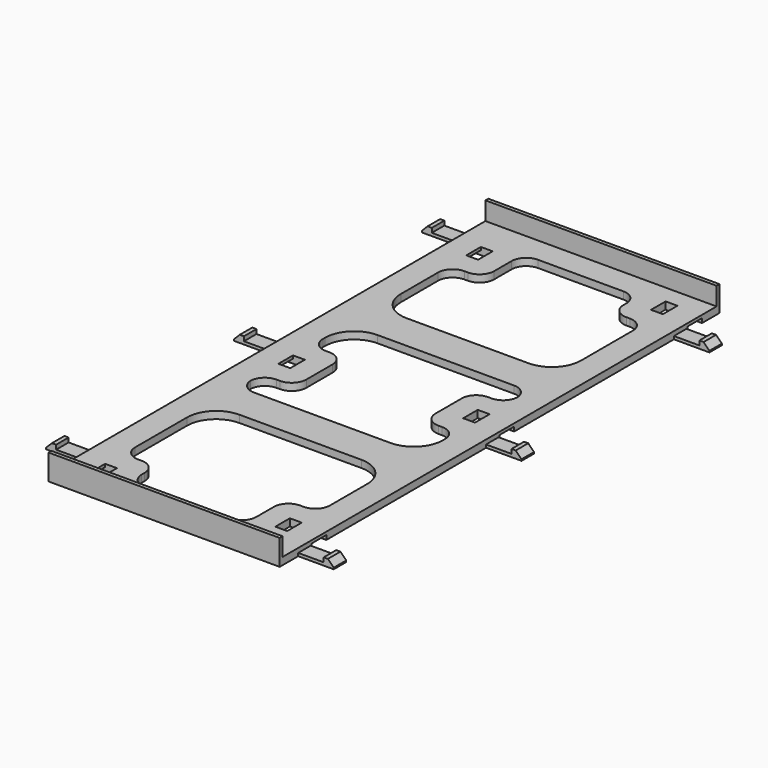
from build123d import *

# Parameters (mm, degrees)
F0_W         = 63.5
F0_H         = 151
F1_DEPTH     = 2
F2_W         = 63.5
F2_H         = 1
F3_DEPTH     = 5
F4_W         = 5
F4_H         = 1.2
F5_DEPTH     = 10
F6_W         = 5
F6_H         = 1.2
F7_DEPTH     = 10
F8_W         = 4.3
F8_H         = 0.8
F9_DEPTH     = 9.75
F10_W        = 4.3
F10_H        = 0.8
F11_DEPTH    = 9.75
F12_W        = 2.75
F12_H        = 4.3
F13_DEPTH    = 1.2
F14_W        = 2.75
F14_H        = 4.3
F15_DEPTH    = 1.2
F16_W        = 2.75
F16_H        = 4.3
F17_DEPTH    = 1.2
F18_W        = 2.75
F18_H        = 4.3
F19_DEPTH    = 1.2
F20_W        = 2.75
F20_H        = 4.3
F21_DEPTH    = 1.2
F22_W        = 2.75
F22_H        = 4.3
F23_DEPTH    = 1.2
F28_W        = 3.25
F28_H        = 5
F29_W        = 3.25
F29_H        = 5
F27_W        = 3.25
F27_H        = 5
F26_W        = 3.25
F26_H        = 5
F25_W        = 3.25
F25_H        = 5
F24_W        = 3.25
F24_H        = 5
F30_DEPTH    = 5.801
F31_SIZE     = 1.6
F33_DEPTH    = 2.001
F34_T1_DEPTH = 2
F34_T3_DEPTH = 22
F35_R        = 8


# Not quite as in the source:
# - a fillet or chamfer that OpenCascade refuses, or shapes differently, is made with other operations: its cross-section is extruded or revolved along the edge and cut away or added


with BuildPart() as f1:
    # F0 (on Top) → F1 (new body)
    with BuildSketch(Plane.XY):
        with Locations((31.75, 75.5)):
            Rectangle(F0_W, F0_H)
    extrude(amount=F1_DEPTH)

    # F2 (on face) → F3 (join)
    with BuildSketch(Plane.XY.offset(2)):
        with Locations((31.75, 0.5)):
            Rectangle(F2_W, F2_H)
        with Locations((31.75, 150.5)):
            Rectangle(F2_W, F2_H)
    extrude(amount=F3_DEPTH)

    # F4 (on face) → F5 (cut)
    with BuildSketch(Plane.YZ.offset(63.5)):
        with Locations((13.5, 0.6)):
            Rectangle(F4_W, F4_H)
        with Locations((78, 0.6)):
            Rectangle(F4_W, F4_H)
        with Locations((142.5, 0.6)):
            Rectangle(F4_W, F4_H)
    extrude(amount=-F5_DEPTH, mode=Mode.SUBTRACT)

    # F6 (on face) → F7 (cut)
    with BuildSketch(Plane(origin=(0, 0, 0), x_dir=(0, -1, 0), z_dir=(-1, 0, 0))):
        with Locations((-137.5, 0.6)):
            Rectangle(F6_W, F6_H)
        with Locations((-73, 0.6)):
            Rectangle(F6_W, F6_H)
        with Locations((-8.5, 0.6)):
            Rectangle(F6_W, F6_H)
    extrude(amount=-F7_DEPTH, mode=Mode.SUBTRACT)

    # F8 (on face) → F9 (join)
    with BuildSketch(Plane.YZ.offset(63.5)):
        with Locations((137.5, 0.4)):
            Rectangle(F8_W, F8_H)
        with Locations((73, 0.4)):
            Rectangle(F8_W, F8_H)
        with Locations((8.5, 0.4)):
            Rectangle(F8_W, F8_H)
    extrude(amount=F9_DEPTH)

    # F10 (on face) → F11 (join)
    with BuildSketch(Plane(origin=(0, 0, 0), x_dir=(0, -1, 0), z_dir=(-1, 0, 0))):
        with Locations((-13.5, 0.4)):
            Rectangle(F10_W, F10_H)
        with Locations((-78, 0.4)):
            Rectangle(F10_W, F10_H)
        with Locations((-142.5, 0.4)):
            Rectangle(F10_W, F10_H)
    extrude(amount=F11_DEPTH)

    # F12 (on face) → F13 (join)
    with BuildSketch(Plane.XY.offset(0.8)):
        with Locations((71.875, 8.5)):
            Rectangle(F12_W, F12_H)
    extrude(amount=F13_DEPTH)

    # F14 (on face) → F15 (join)
    with BuildSketch(Plane.XY.offset(0.8)):
        with Locations((-8.375, 13.5)):
            Rectangle(F14_W, F14_H)
    extrude(amount=F15_DEPTH)

    # F16 (on face) → F17 (join)
    with BuildSketch(Plane.XY.offset(0.8)):
        with Locations((71.875, 73)):
            Rectangle(F16_W, F16_H)
    extrude(amount=F17_DEPTH)

    # F18 (on face) → F19 (join)
    with BuildSketch(Plane.XY.offset(0.8)):
        with Locations((-8.375, 78)):
            Rectangle(F18_W, F18_H)
    extrude(amount=F19_DEPTH)

    # F20 (on face) → F21 (join)
    with BuildSketch(Plane.XY.offset(0.8)):
        with Locations((71.875, 137.5)):
            Rectangle(F20_W, F20_H)
    extrude(amount=F21_DEPTH)

    # F22 (on face) → F23 (join)
    with BuildSketch(Plane.XY.offset(0.8)):
        with Locations((-8.375, 142.5)):
            Rectangle(F22_W, F22_H)
    extrude(amount=F23_DEPTH)

    # F28 (on face) + F29 (on face) + F27 (on face) + F26 (on face) + F25 (on face) + F24 (on face) → F30 (cut, through all)
    with BuildSketch(Plane(origin=(0, 0, 1.2), x_dir=(1, 0, 0), z_dir=(0, 0, -1))):
        with Locations((55.125, -13.5)):
            Rectangle(F28_W, F28_H)
    with BuildSketch(Plane(origin=(0, 0, 1.2), x_dir=(1, 0, 0), z_dir=(0, 0, -1))):
        with Locations((8.375, -8.5)):
            Rectangle(F29_W, F29_H)
    with BuildSketch(Plane(origin=(0, 0, 1.2), x_dir=(1, 0, 0), z_dir=(0, 0, -1))):
        with Locations((8.375, -73)):
            Rectangle(F27_W, F27_H)
    with BuildSketch(Plane(origin=(0, 0, 1.2), x_dir=(1, 0, 0), z_dir=(0, 0, -1))):
        with Locations((55.125, -78)):
            Rectangle(F26_W, F26_H)
    with BuildSketch(Plane(origin=(0, 0, 1.2), x_dir=(1, 0, 0), z_dir=(0, 0, -1))):
        with Locations((8.375, -137.5)):
            Rectangle(F25_W, F25_H)
    with BuildSketch(Plane(origin=(0, 0, 1.2), x_dir=(1, 0, 0), z_dir=(0, 0, -1))):
        with Locations((55.125, -142.5)):
            Rectangle(F24_W, F24_H)
    extrude(amount=-F30_DEPTH, mode=Mode.SUBTRACT)

    # F31
    f31_edges = [f1.edges().sort_by_distance(p)[0] for p in [
        (73.25, 8.5, 2),
        (73.25, 73, 2),
        (73.25, 137.5, 2),
        (-9.75, 142.5, 2),
        (-9.75, 78, 2),
        (-9.75, 13.5, 2),
    ]]
    chamfer(f31_edges, length=F31_SIZE)

    # F32 (on face) → F33 (cut, through all)
    with BuildSketch(Plane.XY.offset(2)):
        Polygon((7, 129), (7, 104.2), (56.5, 104.2), (56.5, 134), (47.5, 134), (47.5, 143), (16, 143), (16, 129), align=None)
        Polygon((7, 64.5), (7, 56.8), (56.5, 56.8), (56.5, 69.5), (47.5, 69.5), (47.5, 86.4947894041), (56.5, 86.4947894041), (56.5, 94.2), (7, 94.2), (7, 81.4947894041), (16, 81.4947894041), (16, 64.5), align=None)
        Polygon((7, 46.8), (7, 17), (16, 17), (16, 8), (47.5, 8), (47.5, 22), (56.5, 22), (56.5, 46.8), align=None)
    extrude(amount=-F33_DEPTH, mode=Mode.SUBTRACT)

    # F34: fillet of radius 4 on 22 edges, made by hand

    # F34_s2 → F34_t1 (join)
    with BuildSketch(Plane.XY):
        with BuildLine():
            ThreePointArc((20, 143), (17.1715728753, 141.8284271247), (16, 139))
            Line((16, 139), (16, 143))
            Line((16, 143), (20, 143))
        make_face()
        with BuildLine():
            ThreePointArc((7, 125), (8.1715728753, 127.8284271247), (11, 129))
            Line((11, 129), (7, 129))
            Line((7, 129), (7, 125))
        make_face()
        with BuildLine():
            ThreePointArc((7, 60.5), (8.1715728753, 63.3284271247), (11, 64.5))
            Line((11, 64.5), (7, 64.5))
            Line((7, 64.5), (7, 60.5))
        make_face()
        with BuildLine():
            ThreePointArc((52.5, 86.4947894041), (55.3284271247, 87.6663622794), (56.5, 90.4947894041))
            Line((56.5, 90.4947894041), (56.5, 86.4947894041))
            Line((56.5, 86.4947894041), (52.5, 86.4947894041))
        make_face()
        with BuildLine():
            ThreePointArc((52.5, 22), (55.3284271247, 23.1715728753), (56.5, 26))
            Line((56.5, 26), (56.5, 22))
            Line((56.5, 22), (52.5, 22))
        make_face()
        with BuildLine():
            ThreePointArc((43.5, 8), (46.3284271247, 9.1715728753), (47.5, 12))
            Line((47.5, 12), (47.5, 8))
            Line((47.5, 8), (43.5, 8))
        make_face()
        with BuildLine():
            ThreePointArc((56.5, 65.5), (55.3284271247, 68.3284271247), (52.5, 69.5))
            Line((52.5, 69.5), (56.5, 69.5))
            Line((56.5, 69.5), (56.5, 65.5))
        make_face()
        with BuildLine():
            ThreePointArc((56.5, 130), (55.3284271247, 132.8284271247), (52.5, 134))
            Line((52.5, 134), (56.5, 134))
            Line((56.5, 134), (56.5, 130))
        make_face()
        with BuildLine():
            ThreePointArc((47.5, 139), (46.3284271247, 141.8284271247), (43.5, 143))
            Line((43.5, 143), (47.5, 143))
            Line((47.5, 143), (47.5, 139))
        make_face()
        with BuildLine():
            ThreePointArc((7, 85.4947894041), (8.1715728753, 82.6663622794), (11, 81.4947894041))
            Line((11, 81.4947894041), (7, 81.4947894041))
            Line((7, 81.4947894041), (7, 85.4947894041))
        make_face()
        with BuildLine():
            ThreePointArc((7, 21), (8.1715728753, 18.1715728753), (11, 17))
            Line((11, 17), (7, 17))
            Line((7, 17), (7, 21))
        make_face()
        with BuildLine():
            ThreePointArc((7, 60.8), (8.1715728753, 57.9715728753), (11, 56.8))
            Line((11, 56.8), (7, 56.8))
            Line((7, 56.8), (7, 60.8))
        make_face()
        with BuildLine():
            ThreePointArc((56.5, 90.2), (55.3284271247, 93.0284271247), (52.5, 94.2))
            Line((52.5, 94.2), (56.5, 94.2))
            Line((56.5, 94.2), (56.5, 90.2))
        make_face()
        with BuildLine():
            ThreePointArc((16, 12), (17.1715728753, 9.1715728753), (20, 8))
            Line((20, 8), (16, 8))
            Line((16, 8), (16, 12))
        make_face()
    extrude(amount=F34_T1_DEPTH)

    # F34_s4 → F34_t3 (cut)
    with BuildSketch(Plane.XY.offset(-10)):
        with BuildLine():
            ThreePointArc((16, 133), (14.8284271247, 130.1715728753), (12, 129))
            Line((12, 129), (16, 129))
            Line((16, 129), (16, 133))
        make_face()
        with BuildLine():
            ThreePointArc((51.5, 134), (48.6715728753, 135.1715728753), (47.5, 138))
            Line((47.5, 138), (47.5, 134))
            Line((47.5, 134), (51.5, 134))
        make_face()
        with BuildLine():
            ThreePointArc((51.5, 69.5), (48.6715728753, 70.6715728753), (47.5, 73.5))
            Line((47.5, 73.5), (47.5, 69.5))
            Line((47.5, 69.5), (51.5, 69.5))
        make_face()
        with BuildLine():
            ThreePointArc((12, 81.4947894041), (14.8284271247, 80.3232165289), (16, 77.4947894041))
            Line((16, 77.4947894041), (16, 81.4947894041))
            Line((16, 81.4947894041), (12, 81.4947894041))
        make_face()
        with BuildLine():
            ThreePointArc((16, 68.5), (14.8284271247, 65.6715728753), (12, 64.5))
            Line((12, 64.5), (16, 64.5))
            Line((16, 64.5), (16, 68.5))
        make_face()
        with BuildLine():
            ThreePointArc((12, 17), (14.8284271247, 15.8284271247), (16, 13))
            Line((16, 13), (16, 17))
            Line((16, 17), (12, 17))
        make_face()
        with BuildLine():
            ThreePointArc((47.5, 82.4947894041), (48.6715728753, 85.3232165289), (51.5, 86.4947894041))
            Line((51.5, 86.4947894041), (47.5, 86.4947894041))
            Line((47.5, 86.4947894041), (47.5, 82.4947894041))
        make_face()
        with BuildLine():
            ThreePointArc((47.5, 18), (48.6715728753, 20.8284271247), (51.5, 22))
            Line((51.5, 22), (47.5, 22))
            Line((47.5, 22), (47.5, 18))
        make_face()
    extrude(amount=F34_T3_DEPTH, mode=Mode.SUBTRACT)

    # F35
    f35_edges = [f1.edges().sort_by_distance(p)[0] for p in [
        (7, 94.2, 1),
        (7, 46.8, 1),
        (56.5, 104.2, 1),
        (56.5, 56.8, 1),
        (7, 104.2, 1),
        (56.5, 46.8, 1),
    ]]
    fillet(f35_edges, radius=F35_R)


solid = f1.part
